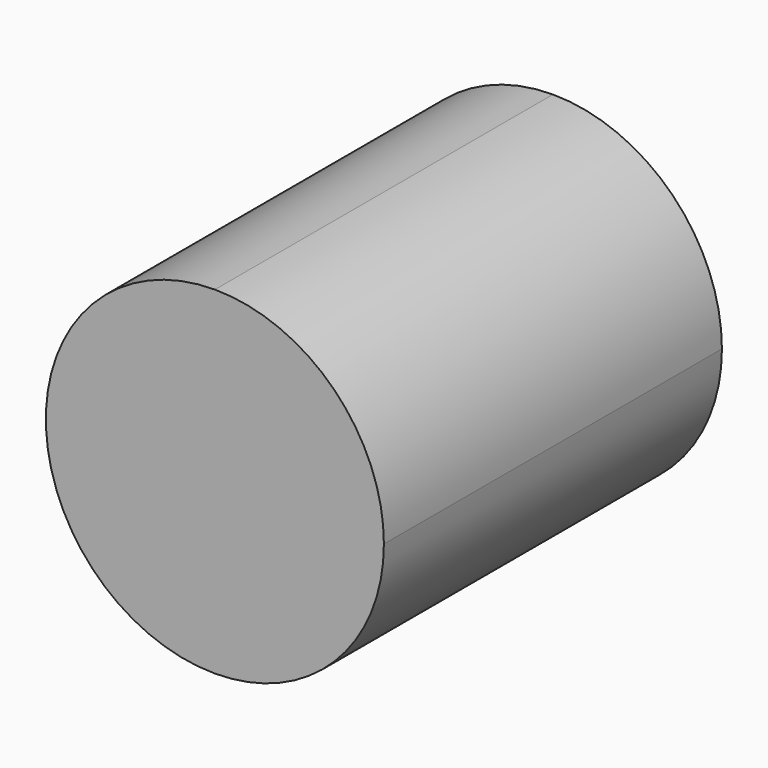
from build123d import *

# Parameters (mm, degrees)
F1_DEPTH = 1.27


# Not quite as in the source:
# - a feature names something its author has since deleted; it is built from what else it names


with BuildPart() as f1:
    # F0 (on Front) → F1 (new body)
    with BuildSketch(Plane.XZ):
        with BuildLine():
            ThreePointArc((0, -0.508), (0.3592102448, -0.3592102448), (0.508, 0))
            ThreePointArc((0.508, 0), (0.3592102448, 0.3592102448), (0, 0.508))
            Line((0, 0.508), (0, 0))
            Line((0, 0), (0, -0.508))
        make_face()
        with BuildLine():
            Line((0, 0), (0, 0.508))
            ThreePointArc((0, 0.508), (-0.508, 0), (0, -0.508))
            Line((0, -0.508), (0, 0))
        make_face()
    extrude(amount=F1_DEPTH)


solid = f1.part
